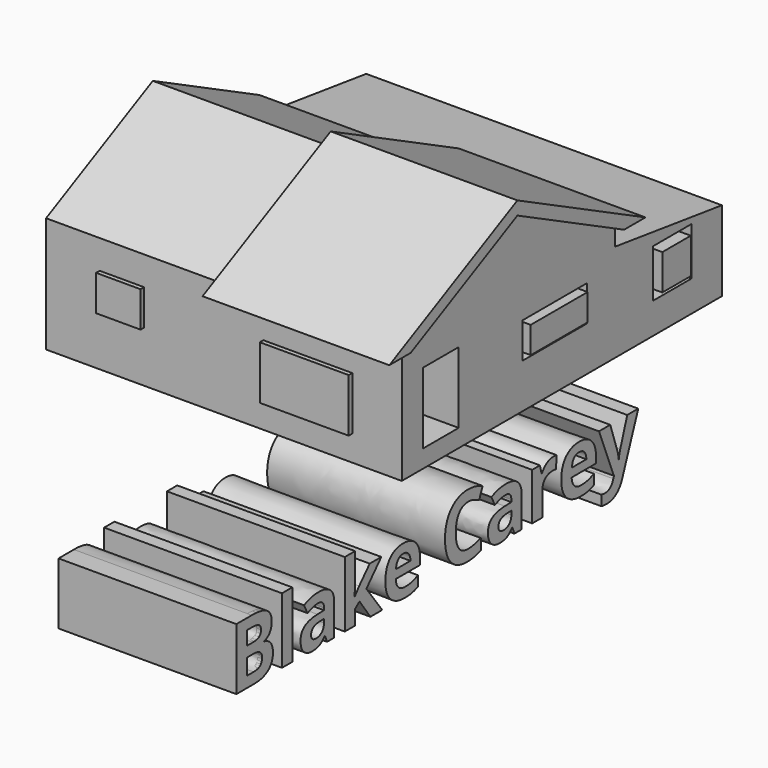
from build123d import *

# Parameters (mm, degrees)
F0_W         = 228.6
F0_H         = 101.6
F0_W_2       = 137.16
F0_H_2       = 137.16
F0_W_3       = 381
F0_H_3       = 50.8
F1_DEPTH     = 508
F2_DEPTH     = 533.4
F0_W_4       = 203.2
F0_H_4       = 76.2
F3_DEPTH     = 520.7
F0_W_5       = 101.6
F4_W         = 127
F4_H         = 101.6
F4_W_2       = 254
F4_H_2       = 152.4
F5_DEPTH     = 12.7
F6_TEXT_SIZE = 246.6833839814
F7_DEPTH     = 508
F0_W_6       = 76.2
F0_H_5       = 177.8
F8_DEPTH     = 12.7


# Not quite as in the source:
# - Text() gives the source's letters only with a copy of the font that has no kerning and outlines rounded to 1/6400 em; it was checked with that copy


with BuildPart() as f1:
    # F0 (on Right) → F1 (new body, symmetric)
    with BuildSketch(Plane.YZ):
        Polygon((-381, 0), (0, 0), (0, 190.5), align=None)
        Polygon((0, 190.5), (0, 0), (381, 0), align=None)
        Polygon((381, 0), (0, 0), (-381, 0), (-381, -279.4), (-304.8, -279.4), (-304.8, -76.2), (-177.8, -76.2), (-177.8, -279.4), (381, -279.4), (381, -50.8), align=None)
        with Locations((165.1, -152.4)):
            Rectangle(F0_W, F0_H, mode=Mode.SUBTRACT)
        Polygon((762, -101.6), (381, -50.8), (381, -279.4), (762, -279.4), align=None)
        with Locations((584.2, -173.1695662854)):
            Rectangle(F0_W_2, F0_H_2, mode=Mode.SUBTRACT)
        Polygon((-304.8, -279.4), (-381, -279.4), (-381, -330.2), (381, -330.2), (381, -279.4), (-177.8, -279.4), (-203.2, -279.4), (-279.4, -279.4), align=None)
        with Locations((571.5, -304.8)):
            Rectangle(F0_W_3, F0_H_3)
    extrude(amount=F1_DEPTH, both=True)

    # F0 (on Right) → F2 (join)
    with BuildSketch(Plane.YZ):
        Polygon((-457.2, 0), (-381, 0), (0, 190.5), (0, 228.6), align=None)
        Polygon((0, 190.5), (381, 0), (457.2, 0), (0, 228.6), align=None)
    extrude(amount=F2_DEPTH)

    # F4 (on face) → F5 (join)
    with BuildSketch(Plane.XZ.offset(381)):
        with Locations((-291.4446274042, -133.1745342731)):
            Rectangle(F4_W, F4_H)
        with Locations((239.5156364441, -181.117006588)):
            Rectangle(F4_W_2, F4_H_2)
    extrude(amount=F5_DEPTH)

    # F0 (on Right) + F7_face (on face) → F8 (join)
    with BuildSketch(Plane.YZ):
        with Locations((-241.3, -190.5)):
            Rectangle(F0_W_6, F0_H_5)
    with BuildSketch(Plane(origin=(508, -911.8631846462, -538.2688888304), x_dir=(0, 1, 0), z_dir=(1, 0, 0))):
        with BuildLine():
            Line((-4.9536231521, 88.1146760031), (-59.7635875304, 88.1146760031))
            Line((-59.7635875304, 88.1146760031), (-59.7635875304, -87.9941335924))
            Line((-59.7635875304, -87.9941335924), (6.1085848483, -87.9941335924))
            add(Edge.make_bspline(
                [(6.1085848483, -87.9941335924), (35.9804008773, -87.9941335924), (70.8244288647, -61.0131384694), (70.8244288647, -19.924937325), (55.9848815471, 0.5420746897), (39.2566645708, 4.2808697282)],
                knots=[0, 0, 0, 1, 2, 2.7056, 3.4112, 3.4112, 3.4112], degree=2))
            Line((39.2566645708, 4.2808697282), (39.2566645708, 5.4757423693))
            add(Edge.make_bspline(
                [(39.2566645708, 5.4757423693), (51.5522894912, 7.5185891429), (66.35329253, 27.7543354851), (66.35329253, 66.7996898559), (32.5114157901, 88.1146760031), (-4.9536231521, 88.1146760031)],
                knots=[0, 0, 0, 1, 2, 3.4707317073, 4.9414634146, 4.9414634146, 4.9414634146], degree=2))
        make_face()
        with BuildLine():
            Line((-22.4141814245, -57.1587105947), (-22.4141814245, -11.2524746069))
            Line((-22.4141814245, -11.2524746069), (0.7123858237, -11.2524746069))
            add(Edge.make_bspline(
                [(0.7123858237, -11.2524746069), (32.0103401664, -11.2524746069), (32.0103401664, -45.3641612981), (17.3249699637, -57.1587105947), (1.9072584649, -57.1587105947)],
                knots=[0, 0, 0, 1, 1.5553602812, 2.1107205624, 2.1107205624, 2.1107205624], degree=2))
            Line((1.9072584649, -57.1587105947), (-22.4141814245, -57.1587105947))
        make_face(mode=Mode.SUBTRACT)
        with BuildLine():
            Line((-0.7522967687, 18.3495314708), (-22.4141814245, 18.3495314708))
            Line((-22.4141814245, 18.3495314708), (-22.4141814245, 57.5105186779))
            Line((-22.4141814245, 57.5105186779), (-2.7951435422, 57.5105186779))
            add(Edge.make_bspline(
                [(-2.7951435422, 57.5105186779), (13.2392764165, 57.5105186779), (28.0402794554, 48.7224231235), (28.0402794554, 27.7543354851), (14.4341490577, 18.3495314708), (-0.7522967687, 18.3495314708)],
                knots=[0, 0, 0, 1, 2, 3.0684410646, 4.1368821293, 4.1368821293, 4.1368821293], degree=2))
        make_face(mode=Mode.SUBTRACT)
    extrude(amount=-F8_DEPTH)


with BuildPart() as f3:
    # F0 (on Right) → F3 (new body)
    with BuildSketch(Plane.YZ):
        with Locations((165.1, -152.4)):
            Rectangle(F0_W_4, F0_H_4)
    extrude(amount=F3_DEPTH)


with BuildPart() as f3b:
    # F0 (on Right) → F3, piece 2 (new body)
    with BuildSketch(Plane.YZ):
        with Locations((584.2, -173.1695662854)):
            Rectangle(F0_W_5, F0_H)
    extrude(amount=F3_DEPTH)


with BuildPart() as f7:
    # F6 (on Right) → F7 (new body)
    with BuildSketch(Plane.YZ):
        with Locations((-993.7897324562, -626.2630224228)):
            Text('Blake Carey', F6_TEXT_SIZE, font='Open Sans', font_style=FontStyle.BOLD, text_align=(TextAlign.LEFT, TextAlign.BOTTOM))
    extrude(amount=F7_DEPTH)


solid = Compound([f1.part, f3.part, f3b.part, f7.part])
